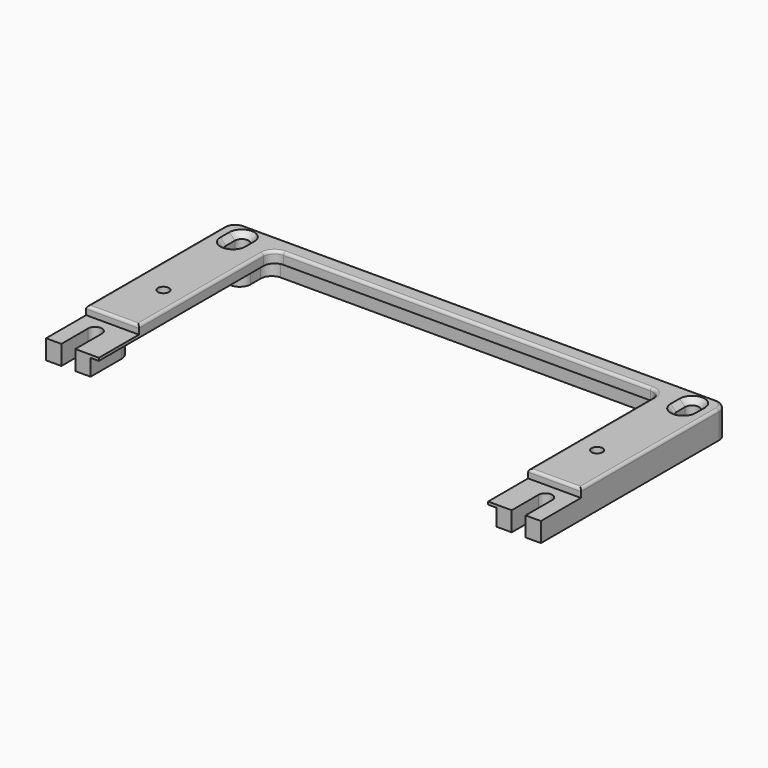
from build123d import *

# Parameters (mm, degrees)
F0_W      = 89
F0_H      = 45
F1_DEPTH  = 5
F2_W      = 70
F2_H      = 39
F3_DEPTH  = 25
F4_W      = 85.5
F4_H      = 41.5
F5_DEPTH  = 3
F6_W      = 8
F6_H      = 8
F6_H_2    = 12
F7_DEPTH  = 3
F8_R      = 1
F9_DEPTH  = 25
F10_DEPTH = 25
F11_W     = 2.5
F11_H     = 2
F12_DEPTH = 25
F13_W     = 89
F13_H     = 3
F14_DEPTH = 25
F15_W     = 89
F15_H     = 9
F16_DEPTH = 1.5
F17_SIZE  = 1
F18_SIZE  = 1
F19_R     = 2
F20_R     = 0.5


with BuildPart() as f1:
    # F0 (on Top) → F1 (new body)
    with BuildSketch(Plane.XY):
        Rectangle(F0_W, F0_H)
    extrude(amount=F1_DEPTH)

    # F2 (on Top) → F3 (cut)
    with BuildSketch(Plane.XY):
        Rectangle(F2_W, F2_H)
    extrude(amount=F3_DEPTH, mode=Mode.SUBTRACT)

    # F4 (on Top) → F5 (cut)
    with BuildSketch(Plane.XY):
        Rectangle(F4_W, F4_H)
    extrude(amount=F5_DEPTH, mode=Mode.SUBTRACT)

    # F6 (on Top) → F7 (join)
    with BuildSketch(Plane.XY):
        with Locations((-40.5, 18.5)):
            Rectangle(F6_W, F6_H)
        with Locations((-40.5, -16.5)):
            Rectangle(F6_W, F6_H_2)
        with Locations((40.5, 18.5)):
            Rectangle(F6_W, F6_H)
        with Locations((40.5, -16.5)):
            Rectangle(F6_W, F6_H_2)
    extrude(amount=F7_DEPTH)

    # F8 (on Top) → F9 (cut)
    with BuildSketch(Plane.XY):
        with BuildLine():
            Line((39.25, -13.5), (41.75, -13.5))
            ThreePointArc((41.75, -13.5), (40.5, -12.25), (39.25, -13.5))
        make_face()
        with BuildLine():
            Line((41.75, -23.5), (41.75, -13.5))
            ThreePointArc((41.75, -13.5), (40.5, -14.75), (39.25, -13.5))
            Line((39.25, -13.5), (39.25, -23.5))
            Line((39.25, -23.5), (41.75, -23.5))
        make_face()
        with BuildLine():
            ThreePointArc((39.25, -13.5), (40.5, -14.75), (41.75, -13.5))
            Line((41.75, -13.5), (39.25, -13.5))
        make_face()
        with BuildLine():
            ThreePointArc((41.25, 18.5), (41.6180339887, 18.9409830056), (41.75, 19.5))
            ThreePointArc((41.75, 19.5), (39.9409830056, 20.6180339887), (39.75, 18.5))
            ThreePointArc((39.75, 18.5), (40.5, 18.75), (41.25, 18.5))
        make_face()
        with BuildLine():
            ThreePointArc((41.25, 18.5), (40.5, 18.75), (39.75, 18.5))
            ThreePointArc((39.75, 18.5), (40.5, 18.25), (41.25, 18.5))
        make_face()
        with BuildLine():
            ThreePointArc((41.25, 18.5), (40.5, 18.25), (39.75, 18.5))
            ThreePointArc((39.75, 18.5), (39.9409830056, 16.3819660113), (41.75, 17.5))
            ThreePointArc((41.75, 17.5), (41.6180339887, 18.0590169944), (41.25, 18.5))
        make_face()
        with BuildLine():
            Line((-41.75, -13.5), (-39.25, -13.5))
            ThreePointArc((-39.25, -13.5), (-40.5, -12.25), (-41.75, -13.5))
        make_face()
        with BuildLine():
            Line((-39.25, -23.5), (-39.25, -13.5))
            ThreePointArc((-39.25, -13.5), (-40.5, -14.75), (-41.75, -13.5))
            Line((-41.75, -13.5), (-41.75, -23.5))
            Line((-41.75, -23.5), (-39.25, -23.5))
        make_face()
        with BuildLine():
            ThreePointArc((-41.75, -13.5), (-40.5, -14.75), (-39.25, -13.5))
            Line((-39.25, -13.5), (-41.75, -13.5))
        make_face()
        with BuildLine():
            ThreePointArc((-39.75, 18.5), (-39.3819660113, 18.9409830056), (-39.25, 19.5))
            ThreePointArc((-39.25, 19.5), (-41.0590169944, 20.6180339887), (-41.25, 18.5))
            ThreePointArc((-41.25, 18.5), (-40.5, 18.75), (-39.75, 18.5))
        make_face()
        with BuildLine():
            ThreePointArc((-39.75, 18.5), (-40.5, 18.75), (-41.25, 18.5))
            ThreePointArc((-41.25, 18.5), (-40.5, 18.25), (-39.75, 18.5))
        make_face()
        with BuildLine():
            ThreePointArc((-39.75, 18.5), (-40.5, 18.25), (-41.25, 18.5))
            ThreePointArc((-41.25, 18.5), (-41.0590169944, 16.3819660113), (-39.25, 17.5))
            ThreePointArc((-39.25, 17.5), (-39.3819660113, 18.0590169944), (-39.75, 18.5))
        make_face()
        with Locations((-39, 0)):
            Circle(F8_R)
        with Locations((39, 0)):
            Circle(F8_R)
    extrude(amount=F9_DEPTH, mode=Mode.SUBTRACT)

    # F8 (on Top) → F10 (cut)
    with BuildSketch(Plane.XY):
        with BuildLine():
            Line((39.25, -13.5), (41.75, -13.5))
            ThreePointArc((41.75, -13.5), (40.5, -12.25), (39.25, -13.5))
        make_face()
        with BuildLine():
            Line((41.75, -23.5), (41.75, -13.5))
            ThreePointArc((41.75, -13.5), (40.5, -14.75), (39.25, -13.5))
            Line((39.25, -13.5), (39.25, -23.5))
            Line((39.25, -23.5), (41.75, -23.5))
        make_face()
        with BuildLine():
            ThreePointArc((39.25, -13.5), (40.5, -14.75), (41.75, -13.5))
            Line((41.75, -13.5), (39.25, -13.5))
        make_face()
        with BuildLine():
            ThreePointArc((41.25, 18.5), (41.6180339887, 18.9409830056), (41.75, 19.5))
            ThreePointArc((41.75, 19.5), (39.9409830056, 20.6180339887), (39.75, 18.5))
            ThreePointArc((39.75, 18.5), (40.5, 18.75), (41.25, 18.5))
        make_face()
        with BuildLine():
            ThreePointArc((41.25, 18.5), (40.5, 18.75), (39.75, 18.5))
            ThreePointArc((39.75, 18.5), (40.5, 18.25), (41.25, 18.5))
        make_face()
        with BuildLine():
            ThreePointArc((41.25, 18.5), (40.5, 18.25), (39.75, 18.5))
            ThreePointArc((39.75, 18.5), (39.9409830056, 16.3819660113), (41.75, 17.5))
            ThreePointArc((41.75, 17.5), (41.6180339887, 18.0590169944), (41.25, 18.5))
        make_face()
        with BuildLine():
            Line((-41.75, -13.5), (-39.25, -13.5))
            ThreePointArc((-39.25, -13.5), (-40.5, -12.25), (-41.75, -13.5))
        make_face()
        with BuildLine():
            Line((-39.25, -23.5), (-39.25, -13.5))
            ThreePointArc((-39.25, -13.5), (-40.5, -14.75), (-41.75, -13.5))
            Line((-41.75, -13.5), (-41.75, -23.5))
            Line((-41.75, -23.5), (-39.25, -23.5))
        make_face()
        with BuildLine():
            ThreePointArc((-41.75, -13.5), (-40.5, -14.75), (-39.25, -13.5))
            Line((-39.25, -13.5), (-41.75, -13.5))
        make_face()
        with BuildLine():
            ThreePointArc((-39.75, 18.5), (-39.3819660113, 18.9409830056), (-39.25, 19.5))
            ThreePointArc((-39.25, 19.5), (-41.0590169944, 20.6180339887), (-41.25, 18.5))
            ThreePointArc((-41.25, 18.5), (-40.5, 18.75), (-39.75, 18.5))
        make_face()
        with BuildLine():
            ThreePointArc((-39.75, 18.5), (-40.5, 18.75), (-41.25, 18.5))
            ThreePointArc((-41.25, 18.5), (-40.5, 18.25), (-39.75, 18.5))
        make_face()
        with BuildLine():
            ThreePointArc((-39.75, 18.5), (-40.5, 18.25), (-41.25, 18.5))
            ThreePointArc((-41.25, 18.5), (-41.0590169944, 16.3819660113), (-39.25, 17.5))
            ThreePointArc((-39.25, 17.5), (-39.3819660113, 18.0590169944), (-39.75, 18.5))
        make_face()
        with Locations((-39, 0)):
            Circle(F8_R)
        with Locations((39, 0)):
            Circle(F8_R)
    extrude(amount=F10_DEPTH, mode=Mode.SUBTRACT)

    # F11 (on face) → F12 (cut)
    with BuildSketch(Plane(origin=(0, 0, 0), x_dir=(1, 0, 0), z_dir=(0, 0, -1))):
        with Locations((-40.5, -18.5)):
            Rectangle(F11_W, F11_H)
        with Locations((40.5, -18.5)):
            Rectangle(F11_W, F11_H)
    extrude(amount=-F12_DEPTH, mode=Mode.SUBTRACT)

    # F13 (on face) → F14 (cut)
    with BuildSketch(Plane.XY.offset(5)):
        with Locations((0, -21)):
            Rectangle(F13_W, F13_H)
    extrude(amount=-F14_DEPTH, mode=Mode.SUBTRACT)

    # F15 (on face) → F16 (cut)
    with BuildSketch(Plane.XY.offset(5)):
        with Locations((0, -15)):
            Rectangle(F15_W, F15_H)
    extrude(amount=-F16_DEPTH, mode=Mode.SUBTRACT)

    # F17
    f17_edges = [f1.edges().sort_by_distance(p)[0] for p in [
        (41.75, 18.5, 5),
    ]]
    chamfer(f17_edges, length=F17_SIZE)

    # F18
    f18_edges = [f1.edges().sort_by_distance(p)[0] for p in [
        (-39.25, 18.5, 5),
    ]]
    chamfer(f18_edges, length=F18_SIZE)

    # F19
    f19_edges = [f1.edges().sort_by_distance(p)[0] for p in [
        (-44.5, 22.5, 2.5),
        (44.5, 22.5, 2.5),
        (35, 19.5, 4),
        (-35, 19.5, 4),
        (-36.5, 14.5, 1.5),
        (-36.5, 20.75, 1.5),
        (-42.75, 14.5, 1.5),
        (-42.75, -10.5, 1.5),
        (-36.5, -10.5, 1.5),
        (36.5, 20.75, 1.5),
        (36.5, 14.5, 1.5),
        (42.75, 14.5, 1.5),
        (42.75, -10.5, 1.5),
        (36.5, -10.5, 1.5),
    ]]
    fillet(f19_edges, radius=F19_R)

    # F20
    f20_edges = [f1.edges().sort_by_distance(p)[0] for p in [
        (0, 22.5, 5),
        (-39.75, -10.5, 5),
        (39.75, -10.5, 5),
        (35, 3.5, 5),
    ]]
    fillet(f20_edges, radius=F20_R)


solid = f1.part
